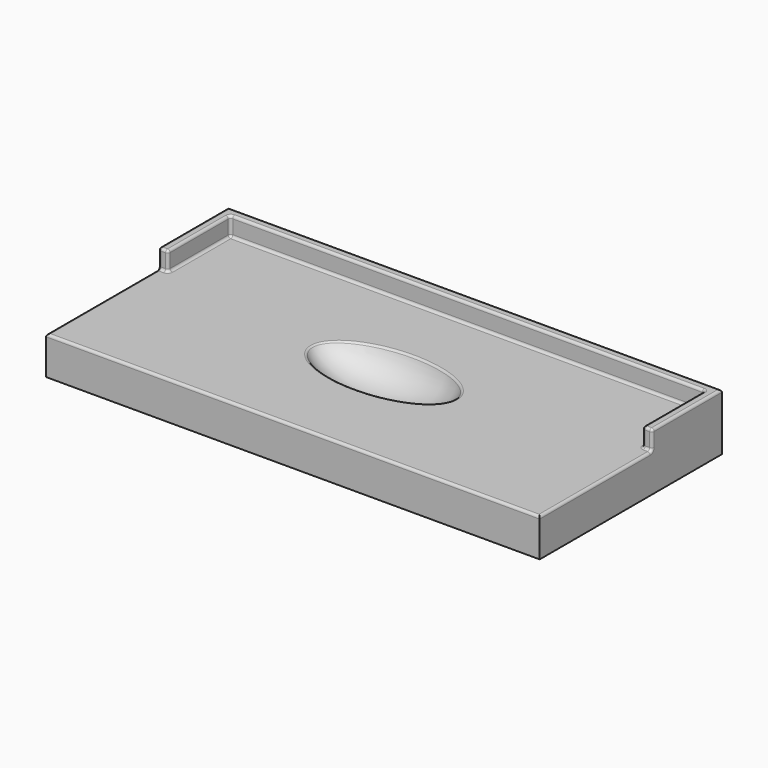
from build123d import *

# Parameters (mm, degrees)
F0_W     = 990.6
F0_H     = 457.2
F1_DEPTH = 76.2
F3_DEPTH = 38.1
F6_R     = 5.08


with BuildPart() as f1:
    # F0 (on Top) → F1 (new body)
    with BuildSketch(Plane.XY):
        Rectangle(F0_W, F0_H)
    extrude(amount=F1_DEPTH)

    # F2 (on face) → F3 (join)
    with BuildSketch(Plane.XY.offset(76.2)):
        Polygon((-495.3, 228.6), (-495.3, 53.6783710122), (-476.25, 53.6783710122), (-476.25, 209.55), (476.25, 209.55), (476.25, 53.6783710122), (495.3, 53.6783710122), (495.3, 228.6), align=None)
    extrude(amount=F3_DEPTH)

    # F4 (on Front) → F5 (revolve, cut)
    with BuildSketch(Plane.XZ):
        with BuildLine():
            Line((152.4, 100.3337353468), (-152.4, 100.3337353468))
            add(Edge.make_bspline(
                [(-152.4, 100.3337353468), (-152.4, 24.1337353468), (0, 24.1337353468), (152.4, 24.1337353468), (152.4, 100.3337353468)],
                knots=[3.1415926536, 3.1415926536, 3.1415926536, 4.7123889804, 4.7123889804, 6.2831853072, 6.2831853072, 6.2831853072], degree=2, weights=[1, 0.7071067812, 1, 0.7071067812, 1]))
        make_face()
    revolve(axis=Axis((0, 0, 100.3337353468), (1, 0, 0)), mode=Mode.SUBTRACT)

    # F6
    f6_edges = [f1.edges().sort_by_distance(p)[0] for p in [
        (495.3, -87.460814, 76.2),
        (485.775, 53.678371, 76.2),
        (476.25, 131.614186, 76.2),
        (0, 209.55, 76.2),
        (-476.25, 131.614186, 76.2),
        (-485.775, 53.678371, 76.2),
        (-495.3, -87.460814, 76.2),
        (0, -228.6, 76.2),
        (144.554527, 0, 76.2),
        (-495.3, 141.139186, 114.3),
        (-485.775, 53.678371, 114.3),
        (-476.25, 131.614186, 114.3),
        (0, 209.55, 114.3),
        (476.25, 131.614186, 114.3),
        (485.775, 53.678371, 114.3),
        (495.3, 141.139186, 114.3),
        (0, 228.6, 114.3),
        (-495.3, 53.678371, 95.25),
        (-476.25, 53.678371, 95.25),
        (-476.25, 209.55, 95.25),
        (476.25, 209.55, 95.25),
        (476.25, 53.678371, 95.25),
        (495.3, 53.678371, 95.25),
    ]]
    fillet(f6_edges, radius=F6_R)


solid = f1.part
